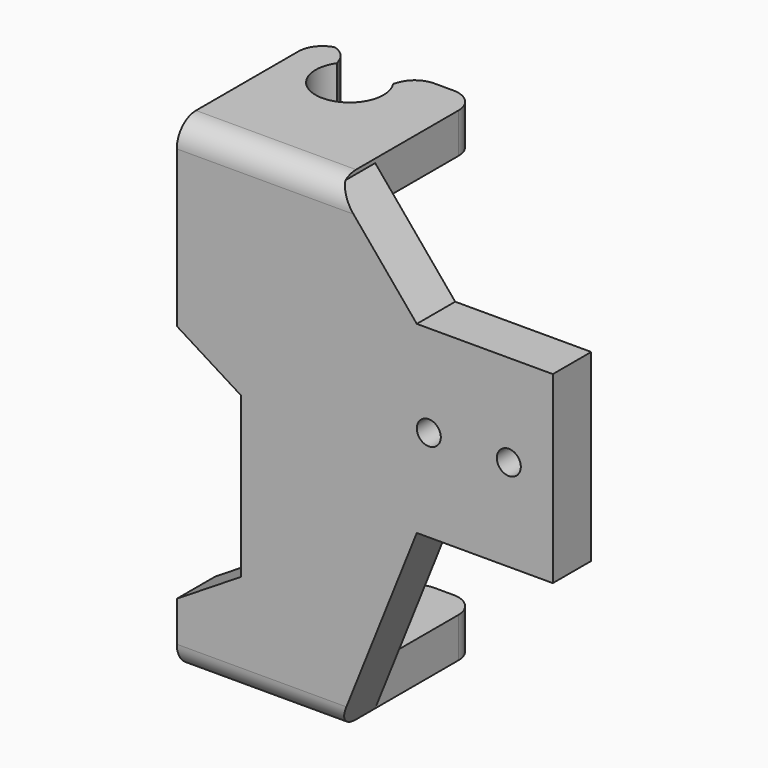
from build123d import *

# Parameters (mm, degrees)
F1_DEPTH    = 20
F3_DEPTH    = 70
F4_R        = 1.5
F5_DEPTH    = 6
F6_T1_DEPTH = 20
F6_T3_DEPTH = 20
F6_T5_DEPTH = 15.2864150343
F6_T7_DEPTH = 15.2864150343
F6_T9_DEPTH = 35
F8_DEPTH    = 25
F9_DEPTH    = 25


# Not quite as in the source:
# - a fillet or chamfer that OpenCascade refuses, or shapes differently, is made with other operations: its cross-section is extruded or revolved along the edge and cut away or added


with BuildPart() as f1:
    # F0 (on Right) → F1 (new body)
    with BuildSketch(Plane.YZ):
        Polygon((0, -26.8219177697), (0, 23.6780822303), (16, 23.6780822303), (16, 28.6780822303), (-6, 28.6780822303), (-6, -31.8219177697), (16, -31.8219177697), (16, -26.8219177697), align=None)
    extrude(amount=F1_DEPTH)

    # F2 (on face) → F3 (cut)
    with BuildSketch(Plane.XY.offset(28.6780822303)):
        with BuildLine():
            ThreePointArc((4.5, 13.4109126902), (6.7375618827, 6.9418292298), (12.25, 11))
            ThreePointArc((12.25, 11), (12.0581707702, 12.2624381173), (11.5, 13.4109126902))
            ThreePointArc((11.5, 13.4109126902), (8, 15.25), (4.5, 13.4109126902))
        make_face()
        with BuildLine():
            ThreePointArc((4.5, 13.4109126902), (8, 15.25), (11.5, 13.4109126902))
            Line((11.5, 13.4109126902), (12.5, 16))
            Line((12.5, 16), (3.5, 16))
            Line((3.5, 16), (4.5, 13.4109126902))
        make_face()
    extrude(amount=-F3_DEPTH, mode=Mode.SUBTRACT)

    # F4 (on face) → F5 (join)
    with BuildSketch(Plane.XZ.offset(6)):
        Polygon((20, 16.1780822303), (20, -6.8219177697), (30, -6.8219177697), (47, -6.8219177697), (47, 16.1780822303), (30, 16.1780822303), align=None)
        with Locations((31.5, 4.6780822303)):
            Circle(F4_R, mode=Mode.SUBTRACT)
        with Locations((41.5, 4.6780822303)):
            Circle(F4_R, mode=Mode.SUBTRACT)
        Polygon((30, -6.8219177697), (20, -6.8219177697), (20, -31.8219177697), align=None)
        Polygon((20, 28.1780822303), (20, 16.1780822303), (30, 16.1780822303), align=None)
    extrude(amount=-F5_DEPTH)

    # F6: fillet of radius 3 on 10 edges, made by hand

    # F6_s2 → F6_t1 (cut)
    with BuildSketch(Plane.XY.offset(16.1780822303)):
        with BuildLine():
            ThreePointArc((17, 16), (19.1213203436, 15.1213203436), (20, 13))
            Line((20, 13), (20, 16))
            Line((20, 16), (17, 16))
        make_face()
        with BuildLine():
            ThreePointArc((0, 13), (0.8786796564, 15.1213203436), (3, 16))
            Line((3, 16), (0, 16))
            Line((0, 16), (0, 13))
        make_face()
    extrude(amount=F6_T1_DEPTH, mode=Mode.SUBTRACT)

    # F6_s4 → F6_t3 (cut)
    with BuildSketch(Plane.XY.offset(-39.3219177697)):
        with BuildLine():
            ThreePointArc((20, 13), (19.1213203436, 15.1213203436), (17, 16))
            Line((17, 16), (20, 16))
            Line((20, 16), (20, 13))
        make_face()
        with BuildLine():
            ThreePointArc((0, 13), (0.8786796564, 15.1213203436), (3, 16))
            Line((3, 16), (0, 16))
            Line((0, 16), (0, 13))
        make_face()
    extrude(amount=F6_T3_DEPTH, mode=Mode.SUBTRACT)

    # F6_s6 → F6_t5 (cut)
    with BuildSketch(Plane.XY.offset(18.5348747132)):
        with BuildLine():
            ThreePointArc((11.7587690029, 14.0808882317), (12.8606193241, 15.4741326455), (14.5572830069, 16))
            Line((14.5572830069, 16), (12.5, 16))
            Line((12.5, 16), (11.7587690029, 14.0808882317))
        make_face()
        with BuildLine():
            ThreePointArc((1.4427169931, 16), (3.1393806759, 15.4741326455), (4.2412309971, 14.0808882317))
            Line((4.2412309971, 14.0808882317), (3.5, 16))
            Line((3.5, 16), (1.4427169931, 16))
        make_face()
    extrude(amount=F6_T5_DEPTH, mode=Mode.SUBTRACT)

    # F6_s8 → F6_t7 (cut)
    with BuildSketch(Plane.XY.offset(-36.9651252868)):
        with BuildLine():
            ThreePointArc((14.5572830069, 16), (12.8606193241, 15.4741326455), (11.7587690029, 14.0808882317))
            Line((11.7587690029, 14.0808882317), (12.5, 16))
            Line((12.5, 16), (14.5572830069, 16))
        make_face()
        with BuildLine():
            ThreePointArc((4.2412309971, 14.0808882317), (3.1393806759, 15.4741326455), (1.4427169931, 16))
            Line((1.4427169931, 16), (3.5, 16))
            Line((3.5, 16), (4.2412309971, 14.0808882317))
        make_face()
    extrude(amount=F6_T7_DEPTH, mode=Mode.SUBTRACT)

    # F6_s10 → F6_t9 (cut)
    with BuildSketch(Plane.YZ.offset(-7.5)):
        with BuildLine():
            ThreePointArc((-3, 28.6780822303), (-5.1213203436, 27.7994025739), (-6, 25.6780822303))
            Line((-6, 25.6780822303), (-6, 28.6780822303))
            Line((-6, 28.6780822303), (-3, 28.6780822303))
        make_face()
        with BuildLine():
            ThreePointArc((-6, -28.8219177697), (-5.1213203436, -30.9432381132), (-3, -31.8219177697))
            Line((-3, -31.8219177697), (-6, -31.8219177697))
            Line((-6, -31.8219177697), (-6, -28.8219177697))
        make_face()
    extrude(amount=F6_T9_DEPTH, mode=Mode.SUBTRACT)

    # F7 (on face) → F8 (cut)
    with BuildSketch(Plane.XZ.offset(6)):
        Polygon((0, 6.1780822303), (0, -23.8219177697), (8, -18.8219177697), (8, 1.1780822303), align=None)
    extrude(amount=-F8_DEPTH, mode=Mode.SUBTRACT)

    # F7 (on face) → F9 (cut)
    with BuildSketch(Plane.XZ.offset(6)):
        Polygon((0, 6.1780822303), (0, -23.8219177697), (8, -18.8219177697), (8, 1.1780822303), align=None)
    extrude(amount=-F9_DEPTH, mode=Mode.SUBTRACT)


solid = f1.part
